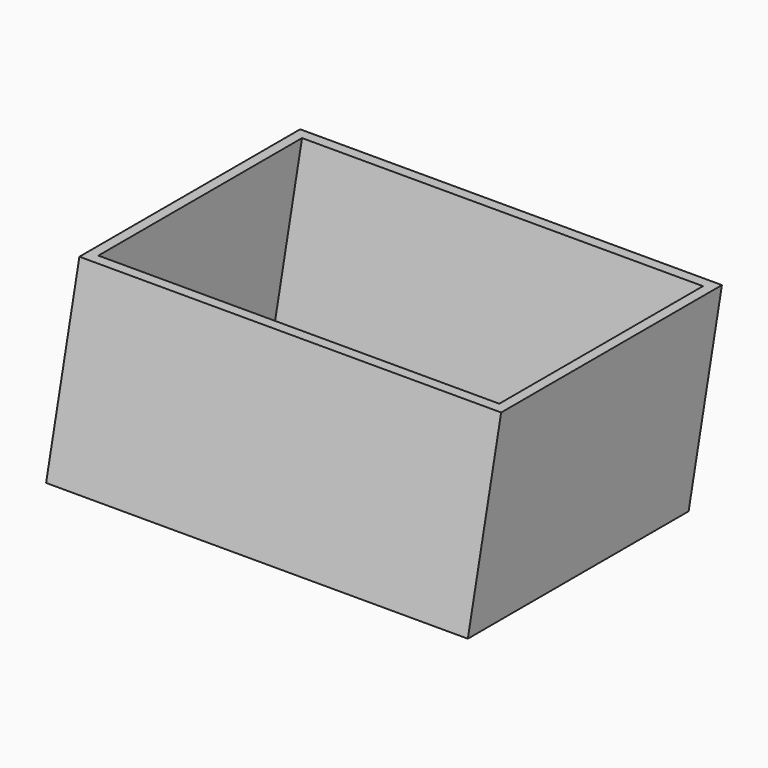
from build123d import *

# Parameters (mm, degrees)
F0_W     = 81
F0_H     = 53
F1_DEPTH = 35
F3_DEPTH = 81
F4_DEPTH = 81.001
F5_T     = -2
F6_DEPTH = 25


with BuildPart() as f1:
    # F0 (on Top) → F1 (new body)
    with BuildSketch(Plane.XY):
        with Locations((6.5364544774, 0)):
            Rectangle(F0_W, F0_H)
    extrude(amount=F1_DEPTH)

    # F2 (on face) → F3 (join, through all)
    with BuildSketch(Plane.YZ.offset(47.0364544774)):
        Polygon((26.5, 35), (26.5, 0), (34.5, 35), align=None)
    extrude(amount=-F3_DEPTH)

    # F2 (on face) → F4 (cut, through all)
    with BuildSketch(Plane.YZ.offset(47.0364544774)):
        Polygon((-26.5, 35), (-26.5, 0), (-18.5, 35), align=None)
    extrude(amount=-F4_DEPTH, mode=Mode.SUBTRACT)

    # F5
    f5_openings = [f1.faces().sort_by_distance(p)[0] for p in [
        (6.536454, 8, 35),
    ]]
    offset(amount=F5_T, openings=f5_openings)

    # F6 (cut): a face of the model
    f6_faces = [f1.faces().sort_by_distance(p)[0] for p in [
        (6.5364544774, 0.4571428571, 2),
    ]]
    extrude(f6_faces, amount=-F6_DEPTH, mode=Mode.SUBTRACT)


solid = f1.part
